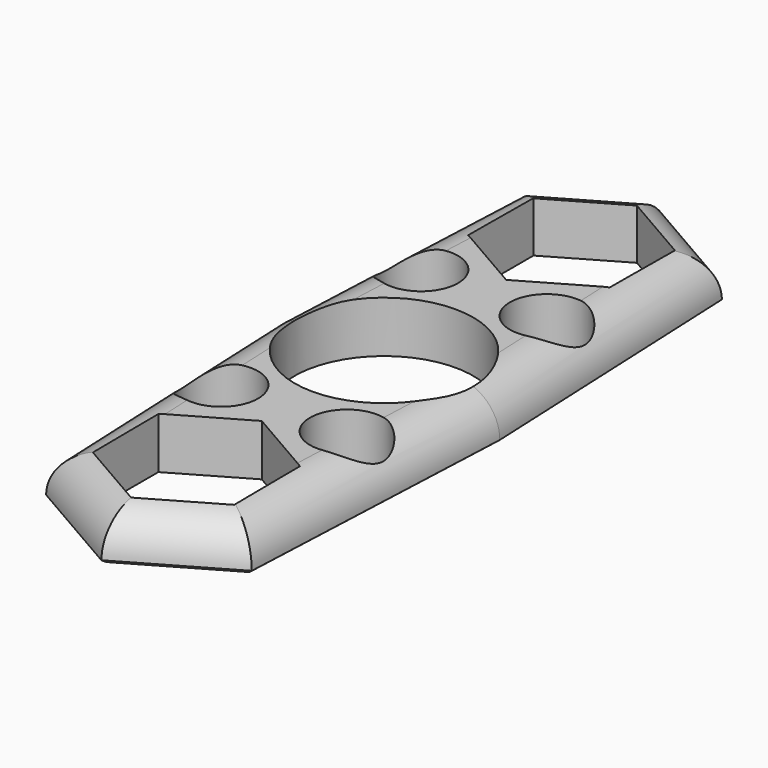
from build123d import *

# Parameters (mm, degrees)
F0_R         = 11.0236
F1_DEPTH     = 6.35
F2_R         = 4.572
F3_DEPTH     = 6.351
F4_T1_DEPTH  = 40.0646968374
F4_T3_DEPTH  = 40.0646968374
F4_T5_DEPTH  = 112.519866921
F4_T7_DEPTH  = 112.519866921
F4_T9_DEPTH  = 40.0646968374
F4_T11_DEPTH = 40.0646968374
F4_T13_DEPTH = 112.519866921
F4_T15_DEPTH = 112.519866921
F5_T1_DEPTH  = 86.7214293968
F5_T3_DEPTH  = 31.4652176625
F5_T5_DEPTH  = 31.4652176625
F5_T7_DEPTH  = 86.7214293968
F5_T9_DEPTH  = 86.7214293968
F5_T11_DEPTH = 31.4652176625
F5_T13_DEPTH = 31.4652176625
F5_T15_DEPTH = 86.7214293968


# Not quite as in the source:
# - a fillet or chamfer that OpenCascade refuses, or shapes differently, is made with other operations: its cross-section is extruded or revolved along the edge and cut away or added


with BuildPart() as f1:
    # F0 (on Top) → F1 (new body)
    with BuildSketch(Plane.XY):
        with BuildLine():
            ThreePointArc((-14.2736051753, -0.6299615453), (-14.2875, -1.804e-07), (-14.2736051912, 0.6299611849))
            Line((-14.2736051912, 0.6299611849), (-14.3014083536, 0))
            Line((-14.3014083536, 0), (-14.2736051753, -0.6299615453))
        make_face()
        with BuildLine():
            ThreePointArc((14.273605172, 0.6299616203), (14.2840258706, 0.3150574191), (14.2875, 0))
            ThreePointArc((14.2875, 0), (14.2840258715, -0.3150573816), (14.2736051753, -0.6299615453))
            Line((14.2736051753, -0.6299615453), (14.3014083536, 0))
            Line((14.3014083536, 0), (14.273605172, 0.6299616203))
        make_face()
        with BuildLine():
            Line((-12.7, -21.6198484187), (0, -14.2875))
            ThreePointArc((0, -14.2875), (-9.8775523454, -10.3231107673), (-14.2736051753, -0.6299615453))
            Line((-14.2736051753, -0.6299615453), (-12.7, -36.2845452561))
            Line((-12.7, -36.2845452561), (-12.7, -21.6198484187))
        make_face()
        with BuildLine():
            Line((12.7, -36.2845452561), (14.2736051753, -0.6299615453))
            ThreePointArc((14.2736051753, -0.6299615453), (9.8775523454, -10.3231107673), (0, -14.2875))
            Line((0, -14.2875), (12.7, -21.6198484187))
            Line((12.7, -21.6198484187), (12.7, -36.2845452561))
        make_face()
        Polygon((-12.7, 21.6198484187), (0, 14.2875), (12.7, 21.6198484187), (12.7, 36.2845452561), (0, 43.6168936748), (-12.7, 36.2845452561), align=None)
        Polygon((0, 18.8628854133), (-8.7376, 23.9075411253), (-8.7376, 33.9968525495), (0, 39.0415082616), (8.7376, 33.9968525495), (8.7376, 23.9075411253), align=None, mode=Mode.SUBTRACT)
        Polygon((12.7, -21.6198484187), (0, -14.2875), (-12.7, -21.6198484187), (-12.7, -36.2845452561), (0, -43.6168936748), (12.7, -36.2845452561), align=None)
        Polygon((-8.7376, -33.9968525495), (-8.7376, -23.9075411253), (0, -18.8628854133), (8.7376, -23.9075411253), (8.7376, -33.9968525495), (0, -39.0415082616), align=None, mode=Mode.SUBTRACT)
        with BuildLine():
            ThreePointArc((14.2736051753, -0.6299615453), (14.2840258715, -0.3150573816), (14.2875, 0))
            ThreePointArc((14.2875, 0), (14.2840258706, 0.3150574191), (14.273605172, 0.6299616203))
            ThreePointArc((14.273605172, 0.6299616203), (9.8775523183, 10.3231107933), (0, 14.2875))
            ThreePointArc((0, 14.2875), (-9.8775524757, 10.3231106426), (-14.2736051912, 0.6299611849))
            ThreePointArc((-14.2736051912, 0.6299611849), (-14.2875, -1.804e-07), (-14.2736051753, -0.6299615453))
            ThreePointArc((-14.2736051753, -0.6299615453), (-9.8775523454, -10.3231107673), (0, -14.2875))
            ThreePointArc((0, -14.2875), (9.8775523454, -10.3231107673), (14.2736051753, -0.6299615453))
        make_face()
        Circle(F0_R, mode=Mode.SUBTRACT)
        with BuildLine():
            ThreePointArc((-14.2736051912, 0.6299611849), (-9.8775524757, 10.3231106426), (0, 14.2875))
            Line((0, 14.2875), (-12.7, 21.6198484187))
            Line((-12.7, 21.6198484187), (-12.7, 36.2845452561))
            Line((-12.7, 36.2845452561), (-14.2736051912, 0.6299611849))
        make_face()
        with BuildLine():
            ThreePointArc((0, 14.2875), (9.8775523183, 10.3231107933), (14.273605172, 0.6299616203))
            Line((14.273605172, 0.6299616203), (12.7, 36.2845452561))
            Line((12.7, 36.2845452561), (12.7, 21.6198484187))
            Line((12.7, 21.6198484187), (0, 14.2875))
        make_face()
    extrude(amount=F1_DEPTH)

    # F2 (on Top) → F3 (cut, through all)
    with BuildSketch(Plane.XY):
        with Locations((-7.7726566461, 15.431494528)):
            Circle(F2_R)
        with Locations((7.7726566461, 15.431494528)):
            Circle(F2_R)
        with Locations((-7.7726566461, -15.431494528)):
            Circle(F2_R)
        with Locations((7.7726566461, -15.431494528)):
            Circle(F2_R)
    extrude(amount=F3_DEPTH, mode=Mode.SUBTRACT)

    # F4: fillet of radius 5.08 on 8 edges, made by hand

    # F4_s2 → F4_t1 (cut)
    with BuildSketch(Plane(origin=(29.8851916063, 17.2542234187, 0), x_dir=(0, 0, 1), z_dir=(-0.8660254038, -0.5, 0))):
        with BuildLine():
            ThreePointArc((6.35, 32.6933379566), (4.8621024484, 36.285440405), (1.27, 37.7733379566))
            Line((1.27, 37.7733379566), (6.35, 37.7733379566))
            Line((6.35, 37.7733379566), (6.35, 32.6933379566))
        make_face()
    extrude(amount=F4_T1_DEPTH, mode=Mode.SUBTRACT)

    # F4_s4 → F4_t3 (cut)
    with BuildSketch(Plane(origin=(4.8118536498, -2.778125, 0), x_dir=(0, 0, 1), z_dir=(-0.8660254038, 0.5, 0))):
        with BuildLine():
            ThreePointArc((6.35, 32.6933379566), (4.8621024484, 36.285440405), (1.27, 37.7733379566))
            Line((1.27, 37.7733379566), (6.35, 37.7733379566))
            Line((6.35, 37.7733379566), (6.35, 32.6933379566))
        make_face()
    extrude(amount=F4_T3_DEPTH, mode=Mode.SUBTRACT)

    # F4_s6 → F4_t5 (cut)
    with BuildSketch(Plane(origin=(2.8276325604, -64.0682068213, 0), x_dir=(0, 0, 1), z_dir=(-0.0440918012, 0.9990274836, 0))):
        with BuildLine():
            ThreePointArc((6.35, 9.2075), (4.8621024484, 12.7996024484), (1.27, 14.2875))
            Line((1.27, 14.2875), (6.35, 14.2875))
            Line((6.35, 14.2875), (6.35, 9.2075))
        make_face()
    extrude(amount=F4_T5_DEPTH, mode=Mode.SUBTRACT)

    # F4_s8 → F4_t7 (cut)
    with BuildSketch(Plane(origin=(-2.1335710483, -48.342232688, 0), x_dir=(0, 0, 1), z_dir=(0.0440918012, 0.9990274836, 0))):
        with BuildLine():
            ThreePointArc((6.35, 9.2075), (4.8621024484, 12.7996024484), (1.27, 14.2875))
            Line((1.27, 14.2875), (6.35, 14.2875))
            Line((6.35, 14.2875), (6.35, 9.2075))
        make_face()
    extrude(amount=F4_T7_DEPTH, mode=Mode.SUBTRACT)

    # F4_s10 → F4_t9 (cut)
    with BuildSketch(Plane(origin=(-29.8851916063, -17.2542234187, 0), x_dir=(0, 0, 1), z_dir=(0.8660254038, 0.5, 0))):
        with BuildLine():
            ThreePointArc((6.35, 32.6933379566), (4.8621024484, 36.285440405), (1.27, 37.7733379566))
            Line((1.27, 37.7733379566), (6.35, 37.7733379566))
            Line((6.35, 37.7733379566), (6.35, 32.6933379566))
        make_face()
    extrude(amount=F4_T9_DEPTH, mode=Mode.SUBTRACT)

    # F4_s12 → F4_t11 (cut)
    with BuildSketch(Plane(origin=(-4.8118536498, 2.778125, 0), x_dir=(0, 0, 1), z_dir=(0.8660254038, -0.5, 0))):
        with BuildLine():
            ThreePointArc((1.27, 37.7733379566), (4.8621024484, 36.285440405), (6.35, 32.6933379566))
            Line((6.35, 32.6933379566), (6.35, 37.7733379566))
            Line((6.35, 37.7733379566), (1.27, 37.7733379566))
        make_face()
    extrude(amount=F4_T11_DEPTH, mode=Mode.SUBTRACT)

    # F4_s14 → F4_t13 (cut)
    with BuildSketch(Plane(origin=(-2.8276325604, 64.0682068213, 0), x_dir=(0, 0, 1), z_dir=(0.0440918012, -0.9990274836, 0))):
        with BuildLine():
            ThreePointArc((1.27, 14.2875), (4.8621024484, 12.7996024484), (6.35, 9.2075))
            Line((6.35, 9.2075), (6.35, 14.2875))
            Line((6.35, 14.2875), (1.27, 14.2875))
        make_face()
    extrude(amount=F4_T13_DEPTH, mode=Mode.SUBTRACT)

    # F4_s16 → F4_t15 (cut)
    with BuildSketch(Plane(origin=(2.1335710483, 48.342232688, 0), x_dir=(0, 0, 1), z_dir=(-0.0440918012, -0.9990274836, 0))):
        with BuildLine():
            ThreePointArc((1.27, 14.2875), (4.8621024484, 12.7996024484), (6.35, 9.2075))
            Line((6.35, 9.2075), (6.35, 14.2875))
            Line((6.35, 14.2875), (1.27, 14.2875))
        make_face()
    extrude(amount=F4_T15_DEPTH, mode=Mode.SUBTRACT)

    # F5: fillet of radius 5.08 on 8 edges, made by hand

    # F5_s2 → F5_t1 (cut)
    with BuildSketch(Plane(origin=(1.8797162439, -42.59041672, 0), x_dir=(0, 0, 1), z_dir=(-0.0440918012, 0.9990274836, 0))):
        with BuildLine():
            ThreePointArc((0, 10.9273958349), (0.3280951188, 12.7234470592), (1.27, 14.2875))
            Line((1.27, 14.2875), (0, 14.2875))
            Line((0, 14.2875), (0, 10.9273958349))
        make_face()
    extrude(amount=F5_T1_DEPTH, mode=Mode.SUBTRACT)

    # F5_s4 → F5_t3 (cut)
    with BuildSketch(Plane(origin=(1.0881699374, -0.6282552063, 0), x_dir=(0, 0, 1), z_dir=(-0.8660254038, 0.5, 0))):
        with BuildLine():
            ThreePointArc((0, 34.4132337915), (0.3280951188, 36.2092850158), (1.27, 37.7733379566))
            Line((1.27, 37.7733379566), (0, 37.7733379566))
            Line((0, 37.7733379566), (0, 34.4132337915))
        make_face()
    extrude(amount=F5_T3_DEPTH, mode=Mode.SUBTRACT)

    # F5_s6 → F5_t5 (cut)
    with BuildSketch(Plane(origin=(26.161507894, 15.104353625, 0), x_dir=(0, 0, 1), z_dir=(-0.8660254038, -0.5, 0))):
        with BuildLine():
            ThreePointArc((0, 34.4132337915), (0.3280951188, 36.2092850158), (1.27, 37.7733379566))
            Line((1.27, 37.7733379566), (0, 37.7733379566))
            Line((0, 37.7733379566), (0, 34.4132337915))
        make_face()
    extrude(amount=F5_T5_DEPTH, mode=Mode.SUBTRACT)

    # F5_s8 → F5_t7 (cut)
    with BuildSketch(Plane(origin=(1.943987785, 44.0466746677, 0), x_dir=(0, 0, 1), z_dir=(-0.0440918012, -0.9990274836, 0))):
        with BuildLine():
            ThreePointArc((0, 10.9273958349), (0.3280951188, 12.7234470592), (1.27, 14.2875))
            Line((1.27, 14.2875), (0, 14.2875))
            Line((0, 14.2875), (0, 10.9273958349))
        make_face()
    extrude(amount=F5_T7_DEPTH, mode=Mode.SUBTRACT)

    # F5_s10 → F5_t9 (cut)
    with BuildSketch(Plane(origin=(-1.8797162439, 42.59041672, 0), x_dir=(0, 0, 1), z_dir=(0.0440918012, -0.9990274836, 0))):
        with BuildLine():
            ThreePointArc((1.27, 14.2875), (0.3280951188, 12.7234470592), (0, 10.9273958349))
            Line((0, 10.9273958349), (0, 14.2875))
            Line((0, 14.2875), (1.27, 14.2875))
        make_face()
    extrude(amount=F5_T9_DEPTH, mode=Mode.SUBTRACT)

    # F5_s12 → F5_t11 (cut)
    with BuildSketch(Plane(origin=(-1.0881699374, 0.6282552063, 0), x_dir=(0, 0, 1), z_dir=(0.8660254038, -0.5, 0))):
        with BuildLine():
            ThreePointArc((0, 34.4132337915), (0.3280951188, 36.2092850158), (1.27, 37.7733379566))
            Line((1.27, 37.7733379566), (0, 37.7733379566))
            Line((0, 37.7733379566), (0, 34.4132337915))
        make_face()
    extrude(amount=F5_T11_DEPTH, mode=Mode.SUBTRACT)

    # F5_s14 → F5_t13 (cut)
    with BuildSketch(Plane(origin=(-26.161507894, -15.104353625, 0), x_dir=(0, 0, 1), z_dir=(0.8660254038, 0.5, 0))):
        with BuildLine():
            ThreePointArc((0, 34.4132337915), (0.3280951188, 36.2092850158), (1.27, 37.7733379566))
            Line((1.27, 37.7733379566), (0, 37.7733379566))
            Line((0, 37.7733379566), (0, 34.4132337915))
        make_face()
    extrude(amount=F5_T13_DEPTH, mode=Mode.SUBTRACT)

    # F5_s16 → F5_t15 (cut)
    with BuildSketch(Plane(origin=(-1.943987785, -44.0466746677, 0), x_dir=(0, 0, 1), z_dir=(0.0440918012, 0.9990274836, 0))):
        with BuildLine():
            ThreePointArc((0, 10.9273958349), (0.3280951188, 12.7234470592), (1.27, 14.2875))
            Line((1.27, 14.2875), (0, 14.2875))
            Line((0, 14.2875), (0, 10.9273958349))
        make_face()
    extrude(amount=F5_T15_DEPTH, mode=Mode.SUBTRACT)


solid = f1.part
